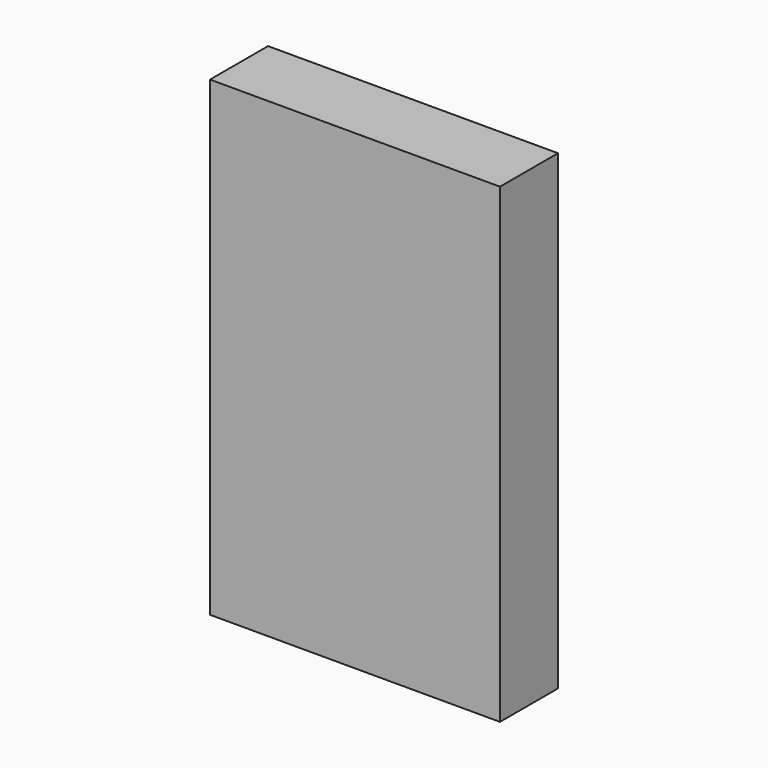
from build123d import *

# Parameters (mm, degrees)
F0_W     = 50.8
F0_H     = 82.55
F1_DEPTH = 12.7


# Not quite as in the source:
# - a feature names something its author has since deleted; it is built from what else it names


with BuildPart() as f1:
    # F0 (on Front) → F1 (new body)
    with BuildSketch(Plane.XZ):
        with Locations((25.4, 0)):
            Rectangle(F0_W, F0_H)
    extrude(amount=F1_DEPTH)


solid = f1.part
